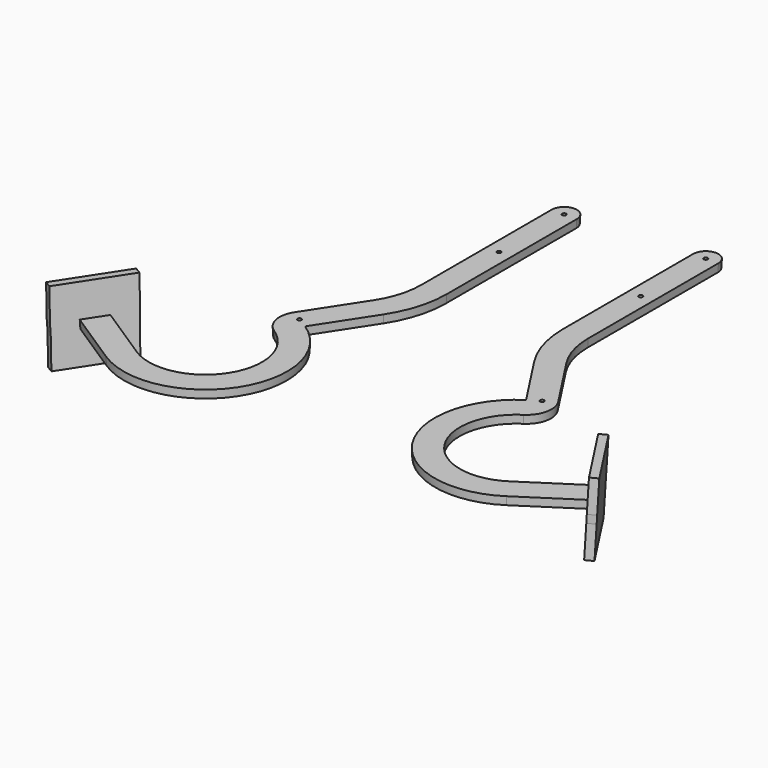
from build123d import *

# Parameters (mm, degrees)
F1_DEPTH                 = 5
DRAFT_F1_DRAFTED_ANGLE   = -3
DRAFT_F1_2_DRAFTED_ANGLE = -3
F3_DEPTH                 = 5
F5_DEPTH                 = 5


# Not quite as in the source:
# - an extrude with a draft is written as a straight extrude whose walls are then drafted


with BuildPart() as f1:
    # F0 (on Top) → F1 (new body)
    with BuildSketch(Plane.XY):
        with BuildLine():
            Line((-38.7264100677, 82.8834338109), (-32.7264100677, 82.8834338109))
            ThreePointArc((-32.7264100677, 82.8834338109), (-40.2264100677, 90.3834338109), (-47.7264100677, 82.8834338109))
            Line((-47.7264100677, 82.8834338109), (-41.7264100677, 82.8834338109))
            ThreePointArc((-41.7264100677, 82.8834338109), (-40.2264100677, 84.3834338109), (-38.7264100677, 82.8834338109))
        make_face()
        with BuildLine():
            Line((-32.7264100677, -17.1165661891), (-32.7264100677, 82.8834338109))
            Line((-32.7264100677, 82.8834338109), (-38.7264100677, 82.8834338109))
            ThreePointArc((-38.7264100677, 82.8834338109), (-39.1657498959, 81.8227736391), (-40.2264100677, 81.3834338109))
            ThreePointArc((-40.2264100677, 81.3834338109), (-41.2870702394, 81.8227736391), (-41.7264100677, 82.8834338109))
            Line((-41.7264100677, 82.8834338109), (-47.7264100677, 82.8834338109))
            Line((-47.7264100677, 82.8834338109), (-47.7264100677, -17.1165661891))
            Line((-47.7264100677, -17.1165661891), (-32.7264100677, -17.1165661891))
        make_face()
        with BuildLine():
            ThreePointArc((-38.7264100677, 32.8834338109), (-41.2870702394, 31.8227736391), (-40.2264100677, 34.3834338109))
            ThreePointArc((-40.2264100677, 34.3834338109), (-39.1657498959, 33.9440939827), (-38.7264100677, 32.8834338109))
        make_face(mode=Mode.SUBTRACT)
        with BuildLine():
            ThreePointArc((-43.157921049, -52.2266447548), (-35.3894313737, -35.4300450929), (-32.7264100677, -17.1165661891))
            Line((-32.7264100677, -17.1165661891), (-47.7264100677, -17.1165661891))
            ThreePointArc((-47.7264100677, -17.1165661891), (-49.7682171099, -31.1579822713), (-55.7245182821, -44.0363679596))
            Line((-55.7245182821, -44.0363679596), (-43.157921049, -52.2266447548))
        make_face()
        with BuildLine():
            Line((-64.9986591696, -85.7375707096), (-43.157921049, -52.2266447548))
            Line((-43.157921049, -52.2266447548), (-55.7245182821, -44.0363679596))
            Line((-55.7245182821, -44.0363679596), (-77.5652564027, -77.5472939144))
            Line((-77.5652564027, -77.5472939144), (-72.5386175095, -80.8234046325))
            ThreePointArc((-72.5386175095, -80.8234046325), (-70.854751504, -80.2045537384), (-69.7819577862, -81.642432312))
            ThreePointArc((-69.7819577862, -81.642432312), (-69.8440792125, -82.0696385942), (-70.0252980629, -82.4614599915))
            Line((-70.0252980629, -82.4614599915), (-64.9986591696, -85.7375707096))
        make_face()
        with BuildLine():
            Line((-73.1889359649, -98.3041679427), (-64.9986591696, -85.7375707096))
            Line((-64.9986591696, -85.7375707096), (-70.0252980629, -82.4614599915))
            ThreePointArc((-70.0252980629, -82.4614599915), (-72.1009854657, -82.8990920353), (-72.5386175095, -80.8234046325))
            Line((-72.5386175095, -80.8234046325), (-77.5652564027, -77.5472939144))
            ThreePointArc((-77.5652564027, -77.5472939144), (-79.6759855513, -88.8320965679), (-73.1889359649, -98.3041679427))
        make_face()
        with BuildLine():
            ThreePointArc((-119.6005044712, -169.5148855966), (-50.4109243769, -154.9271508039), (-64.9986591696, -85.7375707096))
            Line((-64.9986591696, -85.7375707096), (-73.1889359649, -98.3041679427))
            ThreePointArc((-73.1889359649, -98.3041679427), (-62.97752161, -146.7368740086), (-111.4102276759, -156.9482883636))
            Line((-111.4102276759, -156.9482883636), (-119.6005044712, -169.5148855966))
        make_face()
        Polygon((-153.1114304259, -147.674147476), (-119.6005044712, -169.5148855966), (-111.4102276759, -156.9482883636), (-144.9211536307, -135.107550243), align=None)
    extrude(amount=F1_DEPTH)

    # draft_F1_drafted
    draft_f1_drafted_walls = [f1.faces().sort_by_distance(p)[0] for p in [
        (-41.7264100677, 82.8834338109, 3.3333333333),
        (-40.2264100677, 90.3834338109, 3.3333333333),
        (-47.7264100677, 32.8834338109, 3.3333333333),
        (-49.7682171099, -31.1579822713, 3.3333333333),
        (-66.6448873424, -60.791830937, 3.3333333333),
        (-79.6759855513, -88.8320965679, 3.3333333333),
        (-62.97752161, -146.7368740086, 3.3333333333),
        (-128.1656906533, -146.0279193033, 3.3333333333),
        (-149.0162920283, -141.3908488595, 3.3333333333),
        (-136.3559674485, -158.5945165363, 3.3333333333),
        (-50.4109243769, -154.9271508039, 3.3333333333),
        (-54.0782901093, -68.9821077322, 3.3333333333),
        (-35.3894313737, -35.4300450929, 3.3333333333),
        (-32.7264100677, 32.8834338109, 3.3333333333),
        (-72.5386175095, -80.8234046325, 3.3333333333),
        (-40.2264100677, 31.3834338109, 3.3333333333),
    ]]
    draft(draft_f1_drafted_walls, neutral_plane=Plane.XY, angle=DRAFT_F1_DRAFTED_ANGLE)

    # F4 (on face) → F5 (join)
    with BuildSketch(Plane(origin=(-39.8020557719, 25.9409805014, -2.4898594049), x_dir=(-0.544206383, -0.8382603769, -0.0340434019), z_dir=(-0.8366250099, 0.5452701537, -0.0523359562))):
        Polygon((222.1960877807, 15.0835967973), (207.2048063372, 14.5722449789), (191.6897517143, 14.0430272851), (176.6984702709, 13.5316754667), (177.1310413839, 8.5366568483), (177.8128438083, -11.4517184097), (222.7866881388, -9.9176629547), (222.1048857143, 10.0707123033), align=None)
        Polygon((191.6897517143, 14.0430272851), (207.2048063372, 14.5722449789), (222.1960877807, 15.0835967973), (221.5142853562, 35.0719720552), (176.0166678464, 33.5200507247), (176.6984702709, 13.5316754667), align=None)
    extrude(amount=F5_DEPTH)


with BuildPart() as f1_2:
    # F0 (on Top) → F1, piece 2 (new body)
    with BuildSketch(Plane.XY):
        with BuildLine():
            ThreePointArc((49.0319251651, 89.4494442265), (41.5319251651, 96.9494442265), (34.0319251651, 89.4494442265))
            Line((34.0319251651, 89.4494442265), (40.0319251651, 89.4494442265))
            ThreePointArc((40.0319251651, 89.4494442265), (41.5319251651, 90.9494442265), (43.0319251651, 89.4494442265))
            Line((43.0319251651, 89.4494442265), (49.0319251651, 89.4494442265))
        make_face()
        with BuildLine():
            Line((40.0319251651, 89.4494442265), (34.0319251651, 89.4494442265))
            Line((34.0319251651, 89.4494442265), (34.0319251651, -10.5505557735))
            Line((34.0319251651, -10.5505557735), (49.0319251651, -10.5505557735))
            Line((49.0319251651, -10.5505557735), (49.0319251651, 89.4494442265))
            Line((49.0319251651, 89.4494442265), (43.0319251651, 89.4494442265))
            ThreePointArc((43.0319251651, 89.4494442265), (42.5925853369, 88.3887840547), (41.5319251651, 87.9494442265))
            ThreePointArc((41.5319251651, 87.9494442265), (40.4712649933, 88.3887840547), (40.0319251651, 89.4494442265))
        make_face()
        with BuildLine():
            ThreePointArc((43.0319251651, 39.4494442265), (40.4712649933, 38.3887840547), (41.5319251651, 40.9494442265))
            ThreePointArc((41.5319251651, 40.9494442265), (42.5925853369, 40.5101043983), (43.0319251651, 39.4494442265))
        make_face(mode=Mode.SUBTRACT)
        with BuildLine():
            Line((49.0319251651, -10.5505557735), (34.0319251651, -10.5505557735))
            ThreePointArc((34.0319251651, -10.5505557735), (36.6949688103, -28.8640466627), (44.4635203117, -45.6606343393))
            Line((44.4635203117, -45.6606343393), (57.0300814626, -37.4703021823))
            ThreePointArc((57.0300814626, -37.4703021823), (51.0737451363, -24.5919521684), (49.0319251651, -10.5505557735))
        make_face()
        with BuildLine():
            Line((57.0300814626, -37.4703021823), (44.4635203117, -45.6606343393))
            Line((44.4635203117, -45.6606343393), (66.3044060637, -79.1714640749))
            Line((66.3044060637, -79.1714640749), (71.331030524, -75.8953312121))
            ThreePointArc((71.331030524, -75.8953312121), (71.7686534234, -73.8196418814), (73.8443427542, -74.2572647807))
            Line((73.8443427542, -74.2572647807), (78.8709672145, -70.9811319179))
            Line((78.8709672145, -70.9811319179), (57.0300814626, -37.4703021823))
        make_face()
        with BuildLine():
            Line((71.331030524, -75.8953312121), (66.3044060637, -79.1714640749))
            Line((66.3044060637, -79.1714640749), (74.4947382207, -91.7380252258))
            ThreePointArc((74.4947382207, -91.7380252258), (80.981746078, -82.2659252725), (78.8709672145, -70.9811319179))
            Line((78.8709672145, -70.9811319179), (73.8443427542, -74.2572647807))
            ThreePointArc((73.8443427542, -74.2572647807), (74.0255642717, -74.649088547), (74.0876866391, -75.0762979964))
            ThreePointArc((74.0876866391, -75.0762979964), (73.0148960885, -76.514175629), (71.331030524, -75.8953312121))
        make_face()
        with BuildLine():
            Line((74.4947382207, -91.7380252258), (66.3044060637, -79.1714640749))
            ThreePointArc((66.3044060637, -79.1714640749), (51.7169760841, -148.3611084344), (120.9066204435, -162.948538414))
            Line((120.9066204435, -162.948538414), (112.7162882866, -150.3819772631))
            ThreePointArc((112.7162882866, -150.3819772631), (64.2835372349, -140.1707762774), (74.4947382207, -91.7380252258))
        make_face()
        Polygon((112.7162882866, -150.3819772631), (120.9066204435, -162.948538414), (154.4174501792, -141.1076526621), (146.2271180222, -128.5410915112), align=None)
    extrude(amount=F1_DEPTH)

    # draft_F1_2_drafted
    draft_f1_2_drafted_walls = [f1_2.faces().sort_by_distance(p)[0] for p in [
        (41.5319251651, 96.9494442265, 3.3333333333),
        (34.0319251651, 39.4494442265, 3.3333333333),
        (36.6949688103, -28.8640466627, 3.3333333333),
        (55.3839631877, -62.4160492071, 3.3333333333),
        (51.7169760841, -148.3611084344, 3.3333333333),
        (137.6620353114, -152.028095538, 3.3333333333),
        (150.3222841007, -134.8243720866, 3.3333333333),
        (129.4717031544, -139.4615343872, 3.3333333333),
        (64.2835372349, -140.1707762774, 3.3333333333),
        (80.981746078, -82.2659252725, 3.3333333333),
        (67.9505243386, -54.2257170501, 3.3333333333),
        (51.0737451363, -24.5919521684, 3.3333333333),
        (49.0319251651, 39.4494442265, 3.3333333333),
        (71.331030524, -75.8953312121, 3.3333333333),
        (40.0319251651, 89.4494442265, 3.3333333333),
        (40.0319251651, 39.4494442265, 3.3333333333),
    ]]
    draft(draft_f1_2_drafted_walls, neutral_plane=Plane.XY, angle=DRAFT_F1_2_DRAFTED_ANGLE)

    # F2 (on face) → F3 (join)
    with BuildSketch(Plane(origin=(43.7108693738, 28.4888232146, -2.7343871966), x_dir=(-0.5442100555, 0.8382579794, 0.0340437294), z_dir=(0.8366226077, 0.5452738394, -0.0523359562))):
        Polygon((-202.3201449237, 9.6409281084), (-187.328863648, 9.1295713711), (-172.3375823723, 8.6182146337), (-171.9050096203, 13.6132331103), (-171.2232006372, 33.6016081445), (-216.7208176378, 35.1535444038), (-217.4026266209, 15.1651693696), (-217.3114261994, 10.1522848457), align=None)
        Polygon((-172.3375823723, 8.6182146337), (-187.328863648, 9.1295713711), (-202.3201449237, 9.6409281084), (-217.3114261994, 10.1522848457), (-217.9932351825, -9.8360901886), (-173.0193913554, -11.3701604005), align=None)
    extrude(amount=F3_DEPTH)


solid = Compound([f1.part, f1_2.part])
